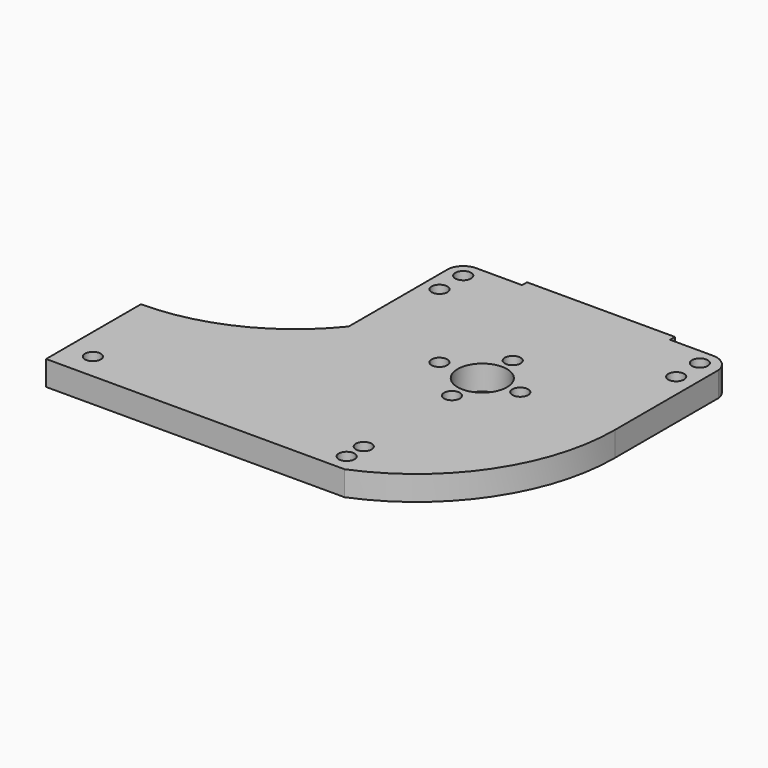
from build123d import *

# Parameters (mm, degrees)
F0_R     = 2.032
F0_R_2   = 2.0279464285
F0_R_3   = 6.35
F1_DEPTH = 6.35


# Not quite as in the source:
# - a feature names something its author has since deleted; it is built from what else it names


with BuildPart() as f1:
    # F0 (on Top) → F1 (new body)
    with BuildSketch(Plane.XY):
        with BuildLine():
            Line((-61.1627068575, -36.5071908827), (-61.1627068575, -43.0169059006))
            Line((-61.1627068575, -43.0169059006), (-61.1627068575, -44.9605127839))
            Line((-61.1627068575, -44.9605127839), (15.7162476502, -44.9605127839))
            ThreePointArc((15.7162476502, -44.9605127839), (38.7853662126, -26.1405440216), (47.4554415236, 2.3411211257))
            Line((47.4554415236, 2.3411211257), (47.4554415236, 4.3248883003))
            Line((47.4554415236, 4.3248883003), (47.4554415236, 35.7800583649))
            ThreePointArc((47.4554415236, 35.7800583649), (45.8046467005, 38.7657690374), (42.6059814887, 39.9524166811))
            Line((42.6059814887, 39.9524166811), (31.5945293048, 39.9524166811))
            Line((31.5945293048, 39.9524166811), (31.5945293048, 41.5436038705))
            Line((31.5945293048, 41.5436038705), (-6.5054706952, 41.5436038705))
            Line((-6.5054706952, 41.5436038705), (-6.5054706952, 39.9524166811))
            Line((-6.5054706952, 39.9524166811), (-18.0521932819, 39.9524166811))
            Line((-18.0521932819, 39.9524166811), (-18.6032061507, 39.9524166811))
            ThreePointArc((-18.6032061507, 39.9524166811), (-21.5619320606, 38.4303826577), (-22.4728391096, 35.2302428284))
            Line((-22.4728391096, 35.2302428284), (-22.4728391096, 4.1078329732))
            ThreePointArc((-22.4728391096, 4.1078329732), (-39.7163433031, -9.5414513084), (-61.1627068575, -14.4091908827))
            Line((-61.1627068575, -14.4091908827), (-61.1627068575, -36.5071908827))
        make_face()
        with Locations((-54.4728634162, -38.2481282619)):
            Circle(F0_R, mode=Mode.SUBTRACT)
        with Locations((12.5428884775, -40.3309306172)):
            Circle(F0_R, mode=Mode.SUBTRACT)
        with Locations((12.5428884775, -34.8417377142)):
            Circle(F0_R_2, mode=Mode.SUBTRACT)
        with Locations((12.5445293048, -6.445995287)):
            Circle(F0_R, mode=Mode.SUBTRACT)
        with Locations((-18.3276997163, 28.1600583649)):
            Circle(F0_R, mode=Mode.SUBTRACT)
        with Locations((-18.3276997163, 35.7800583649)):
            Circle(F0_R, mode=Mode.SUBTRACT)
        with Locations((1.5055636177, 3.3117256275)):
            Circle(F0_R, mode=Mode.SUBTRACT)
        with Locations((12.5445293048, 3.333004713)):
            Circle(F0_R_3, mode=Mode.SUBTRACT)
        with Locations((12.5445293048, 13.112004713)):
            Circle(F0_R, mode=Mode.SUBTRACT)
        with Locations((22.3235293048, 3.333004713)):
            Circle(F0_R, mode=Mode.SUBTRACT)
        with Locations((42.6059814887, 28.1600583649)):
            Circle(F0_R, mode=Mode.SUBTRACT)
        with Locations((42.6059814887, 35.7800583649)):
            Circle(F0_R, mode=Mode.SUBTRACT)
    extrude(amount=F1_DEPTH)


solid = f1.part
